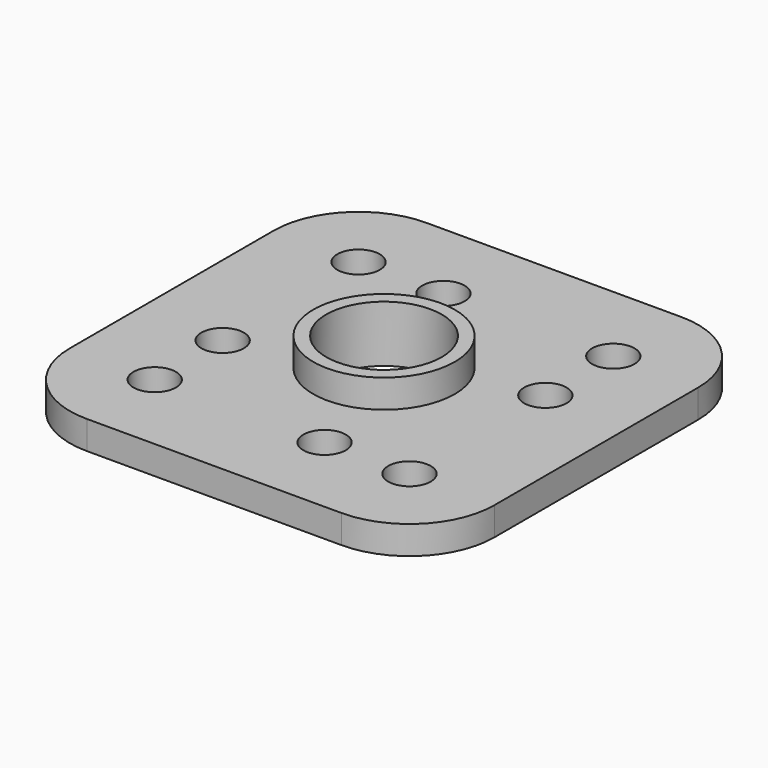
from build123d import *

# Parameters (mm, degrees)
F0_R            = 2.5
F0_R_2          = 2.04
F1_DEPTH        = 1
F2_W            = 15
F2_H            = 15
F2_R            = 5
F2_R_2          = 2.5
F2_R_3          = 2.04
F3_DEPTH        = 1
F4_R            = 3
F5_R            = 0.75
F6_DEPTH        = 25
F6_COPIES_COUNT = 4


# Not quite as in the source:
# - a pattern or mirror of a feature is missing from the dataset's text; its kind, count and spacing are read off the source's solid


with BuildPart() as f1:
    # F0 (on Top) → F1 (new body)
    with BuildSketch(Plane.XY):
        Circle(F0_R)
        Circle(F0_R_2, mode=Mode.SUBTRACT)
    extrude(amount=F1_DEPTH)

    # F2 (on face) → F3 (join)
    with BuildSketch(Plane(origin=(0, 0, 0), x_dir=(1, 0, 0), z_dir=(0, 0, -1))):
        Rectangle(F2_W, F2_H)
        Circle(F2_R, mode=Mode.SUBTRACT)
        Circle(F2_R)
        Circle(F2_R_2, mode=Mode.SUBTRACT)
        Circle(F2_R_2)
        Circle(F2_R_3, mode=Mode.SUBTRACT)
    extrude(amount=F3_DEPTH)

    # F4
    f4_edges = [f1.edges().sort_by_distance(p)[0] for p in [
        (-7.5, 7.5, -0.5),
        (7.5, 7.5, -0.5),
        (-7.5, -7.5, -0.5),
        (7.5, -7.5, -0.5),
    ]]
    fillet(f4_edges, radius=F4_R)

    # F5 (on face) → F6 (cut)
    with BuildSketch(Plane.XY):
        with Locations((-4.5, 4.5)):
            Circle(F5_R)
        with Locations((-1.5, 4.5)):
            Circle(F5_R)
    f6 = extrude(amount=-F6_DEPTH, mode=Mode.SUBTRACT)

    # F6_copies: F6 ×4 about axis
    f6_copies_axis = Axis((0, 0, 0), (0, 0, 1))
    for i in range(1, F6_COPIES_COUNT):
        add(f6.rotate(f6_copies_axis, i * 360 / F6_COPIES_COUNT), mode=Mode.SUBTRACT)


solid = f1.part
